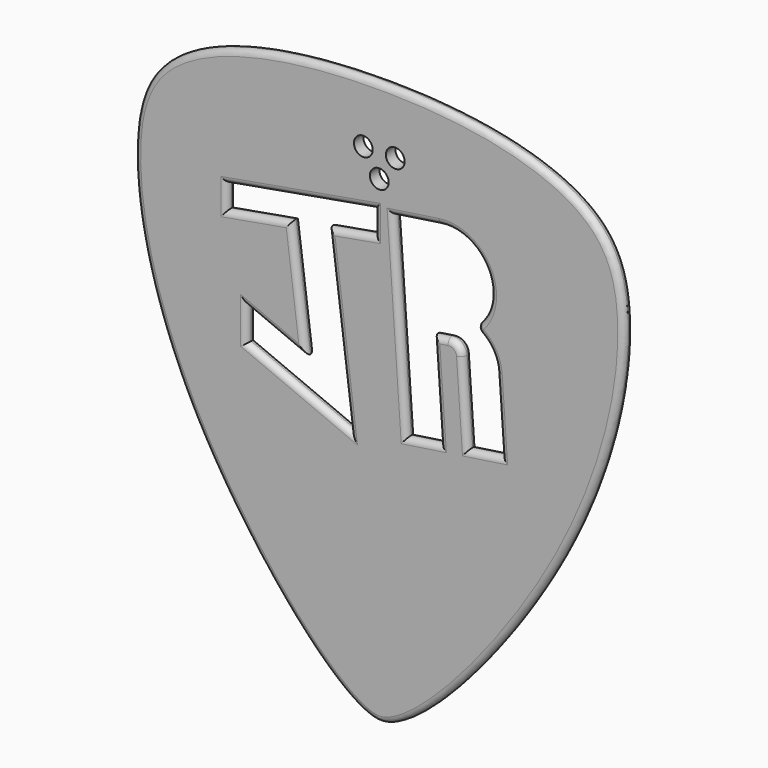
from build123d import *

# Parameters (mm, degrees)
F0_R     = 0.5
F1_DEPTH = 0.63
F2_R     = 0.31499
F3_R     = 0.31499


# Not quite as in the source:
# - a fillet or chamfer is up to 0.001 mm smaller than in the source, because OpenCascade refuses the exact size


with BuildPart() as f1:
    # F0 (on Front) → F1 (new body)
    with BuildSketch(Plane.XZ):
        with BuildLine():
            add(Edge.make_bspline(
                [(0, -23.25), (-2, -23.25), (-11.2052838081, -12.6454945316), (-13.7939030188, -0.3656097413), (-11.4819416014, 5.2828342286), (-5, 6.75), (0, 6.75)],
                knots=[0, 0, 0, 0, 0.2911366771, 0.5724636983, 0.7401439848, 1, 1, 1, 1], degree=3))
            add(Edge.make_bspline(
                [(0, -23.25), (2, -23.25), (11.2052838081, -12.6454945316), (13.7939030188, -0.3656097413), (11.4819416014, 5.2828342286), (5, 6.75), (0, 6.75)],
                knots=[0, 0, 0, 0, 0.2911366771, 0.5724636983, 0.7401439848, 1, 1, 1, 1], degree=3))
        make_face()
        Polygon((-0.25, -0.5), (-2.7097485316, -0.9337200319), (-1.542408067, -10.1097658164), (-7.0756138971, -7.7895000466), (-7.0756138971, -6.0395000466), (-3.9073137099, -7.3680785775), (-4.6816348886, -1.2814167995), (-8.1284620241, -1.8891854213), (-8.1284620241, -0.6391854213), (-0.25, 0.75), align=None, mode=Mode.SUBTRACT)
        with Locations((-0.85, 3.5)):
            Circle(F0_R, mode=Mode.SUBTRACT)
        with BuildLine():
            Line((1.4615160322, -9.4251533127), (0.75, 0.75))
            Line((0.75, 0.75), (3.2225739629, 1.1192939179))
            ThreePointArc((3.2225739629, 1.1192939179), (5.7434258747, -0.2851893969), (5.0276366561, -3.0807060821))
            ThreePointArc((5.0276366561, -3.0807060821), (5.868954756, -3.7604366774), (6.2333425349, -4.7788036907))
            Line((6.2333425349, -4.7788036907), (6.5055669166, -8.6717937201))
            Line((6.5055669166, -8.6717937201), (4.7253136633, -8.937685341))
            Line((4.7253136633, -8.937685341), (4.429349864, -4.7052058231))
            ThreePointArc((4.429349864, -4.7052058231), (4.1692268068, -4.2081365611), (3.6276527318, -4.0617146451))
            Line((3.6276527318, -4.0617146451), (2.8929869168, -4.1714414405))
            Line((2.8929869168, -4.1714414405), (3.2417692855, -9.1592616918))
            Line((3.2417692855, -9.1592616918), (1.4615160322, -9.4251533127))
        make_face(mode=Mode.SUBTRACT)
        with Locations((0, 2.25)):
            Circle(F0_R, mode=Mode.SUBTRACT)
        with BuildLine():
            ThreePointArc((1.35, 3.5), (0.85, 3), (0.35, 3.5))
            ThreePointArc((0.35, 3.5), (0.85, 4), (1.35, 3.5))
        make_face(mode=Mode.SUBTRACT)
    extrude(amount=F1_DEPTH)

    # F2 (radius 0.315 in the source; OpenCascade refuses exactly that, so slightly less here)
    f2_edges = [f1.edges().sort_by_distance(p)[0] for p in [
        (-12.350697, -0.63, -5.69865),
        (12.350697, -0.63, -5.69865),
        (-12.350697, 0, -5.69865),
        (12.350697, 0, -5.69865),
    ]]
    fillet(f2_edges, radius=F2_R)

    # F3 (radius 0.315 in the source; OpenCascade refuses exactly that, so slightly less here)
    f3_edges = [f1.edges().sort_by_distance(p)[0] for p in [
        (-5.491464, -0.63, -6.703789),
        (-4.294474, -0.63, -4.324748),
        (-7.075614, -0.63, -6.9145),
        (-4.309011, -0.63, -8.949633),
        (-2.126078, -0.63, -5.521743),
        (-1.479874, -0.63, -0.71686),
        (-0.25, -0.63, 0.125),
        (-4.189231, -0.63, 0.055407),
        (-8.128462, -0.63, -1.264185),
        (-6.405048, -0.63, -1.585301),
        (1.986287, -0.63, 0.934647),
        (5.743426, -0.63, -0.285189),
        (1.105758, -0.63, -4.337577),
        (2.351643, -0.63, -9.292208),
        (3.067378, -0.63, -6.665352),
        (3.26032, -0.63, -4.116578),
        (5.61544, -0.63, -8.80474),
        (6.369455, -0.63, -6.725299),
        (5.868955, -0.63, -3.760437),
        (5.61544, 0, -8.80474),
        (4.577332, 0, -6.821446),
        (6.369455, 0, -6.725299),
        (5.743426, 0, -0.285189),
        (1.986287, 0, 0.934647),
        (1.105758, 0, -4.337577),
        (3.26032, 0, -4.116578),
        (3.067378, 0, -6.665352),
        (2.351643, 0, -9.292208),
        (-2.126078, 0, -5.521743),
        (-4.309011, 0, -8.949633),
        (-7.075614, 0, -6.9145),
        (-5.491464, 0, -6.703789),
        (-4.294474, 0, -4.324748),
        (-6.405048, 0, -1.585301),
        (-8.128462, 0, -1.264185),
        (-4.189231, 0, 0.055407),
        (-1.479874, 0, -0.71686),
        (-0.25, 0, 0.125),
        (5.027637, -0.315, -3.080706),
    ]]
    fillet(f3_edges, radius=F3_R)


solid = f1.part
